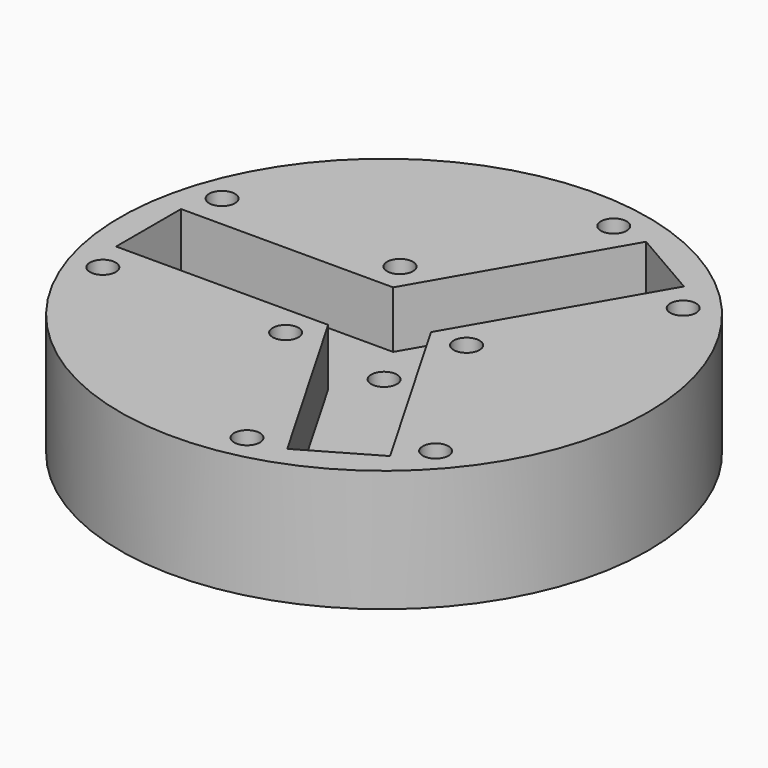
from build123d import *

# Parameters (mm, degrees)
F0_R            = 32.5
F1_DEPTH        = 15
F2_W            = 29
F2_H            = 10
F3_DEPTH        = 7
F3_COPIES_COUNT = 3
F4_R            = 1.5875
F5_DEPTH        = 25.4
F6_R            = 1.5875
F7_DEPTH        = 25.4


# Not quite as in the source:
# - a pattern or mirror of a feature is missing from the dataset's text; its kind, count and spacing are read off the source's solid


with BuildPart() as f1:
    # F0 (on Top) → F1 (new body)
    with BuildSketch(Plane.XY):
        Circle(F0_R)
    extrude(amount=F1_DEPTH)

    # F2 (on face) → F3 (cut)
    with BuildSketch(Plane.XY.offset(15)):
        with Locations((-14.5, 0)):
            Rectangle(F2_W, F2_H)
    f3 = extrude(amount=-F3_DEPTH, mode=Mode.SUBTRACT)

    # F3_copies: F3 ×3 about axis
    f3_copies_axis = Axis((0, 0, 0), (0, 0, 1))
    for i in range(1, F3_COPIES_COUNT):
        add(f3.rotate(f3_copies_axis, i * 360 / F3_COPIES_COUNT), mode=Mode.SUBTRACT)

    # F4 (on face) → F5 (cut)
    with BuildSketch(Plane.XY.offset(8)):
        Circle(F4_R)
    extrude(amount=-F5_DEPTH, mode=Mode.SUBTRACT)

    # F6 (on face) → F7 (cut)
    with BuildSketch(Plane.XY.offset(15)):
        with Locations((10.16, 0)):
            Circle(F6_R)
        with Locations((21.59, 19.05)):
            Circle(F6_R)
        with Locations((21.59, -19.05)):
            Circle(F6_R)
        with Locations((-5.08, 8.7988181024)):
            Circle(F6_R)
        with Locations((5.7027839421, 28.2224884677)):
            Circle(F6_R)
        with Locations((-27.2927839421, 9.1724884677)):
            Circle(F6_R)
        with Locations((-27.2927839421, -9.1724884677)):
            Circle(F6_R)
        with Locations((-5.08, -8.7988181024)):
            Circle(F6_R)
        with Locations((5.7027839421, -28.2224884677)):
            Circle(F6_R)
    extrude(amount=-F7_DEPTH, mode=Mode.SUBTRACT)


solid = f1.part
